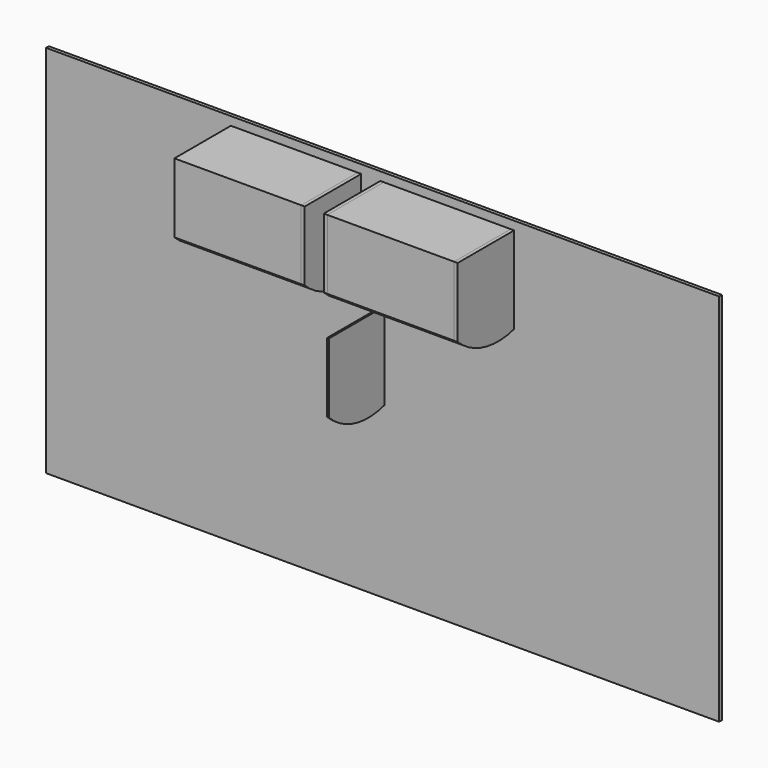
from build123d import *

# Parameters (mm, degrees)
F0_W          = 774.7
F0_H          = 431
F1_DEPTH      = 4
F3_DEPTH      = 2
F3_DEPTH_BACK = 2
F7_DEPTH      = 146
F9_DEPTH      = 2


# Not quite as in the source:
# - a pattern or mirror of a feature is missing from the dataset's text; its kind, count and spacing are read off the source's solid


with BuildPart() as f1:
    # F0 (on Front) → F1 (new body)
    with BuildSketch(Plane.XZ):
        Rectangle(F0_W, F0_H)
    extrude(amount=F1_DEPTH)

    # F8 (on Right) → F9 (join)
    with BuildSketch(Plane.YZ):
        with BuildLine():
            ThreePointArc((-83.8898100026, 0), (-46.6623748041, -21.0902592062), (-3.8898100026, -20))
            Line((-3.8898100026, -20), (-3.8898100026, 80))
            Line((-3.8898100026, 80), (-83.8898100026, 80))
            Line((-83.8898100026, 80), (-83.8898100026, 0))
        make_face()
    extrude(amount=F9_DEPTH)


with BuildPart() as f3:
    # F2 (on Right) → F3 (new body, two sides)
    with BuildSketch(Plane.YZ) as f3_sk:
        with BuildLine():
            ThreePointArc((-86.0752825102, 126.2208398572), (-48.079888449, 105.4589891292), (-4.7887346299, 106.2208398572))
            Line((-4.7887346299, 106.2208398572), (-4.7887346299, 206.2208398572))
            Line((-4.7887346299, 206.2208398572), (-86.0752825102, 206.2208398572))
            Line((-86.0752825102, 206.2208398572), (-86.0752825102, 126.2208398572))
        make_face()
    extrude(amount=F3_DEPTH)
    extrude(f3_sk.sketch, amount=-F3_DEPTH_BACK)


with BuildPart() as f3_copies_1:
    # F3_copies: instance of F3
    add(f3.part.mirror(Plane(origin=(-15, 0, 0), x_dir=(0, 0, -1), z_dir=(-1, 0, 0))))



with BuildPart() as f3_copies1_1:
    # F3_copies1: instance of F3
    add(f3.part.mirror(Plane(origin=(-13, 0, 0), x_dir=(0, 0, -1), z_dir=(-1, 0, 0))))


with BuildPart() as f3_copies2_1:
    # F3_copies2: instance of F3
    add(f3.part.mirror(Plane(origin=(-86, 0, 0), x_dir=(0, 0, -1), z_dir=(-1, 0, 0))))


with BuildPart() as f5_1:
    # F5: instance of F3
    add(f3.part.mirror(Plane.YZ.offset(75)))


with BuildPart() as f7:
    # F7 (new): a face of the model
    f7_faces = [f3.part.faces().sort_by_distance(p)[0] for p in [
        (2, -44.1296538263, 157.155690045),
    ]]
    extrude(f7_faces, amount=F7_DEPTH)


with BuildPart() as f3_copies_1_1:
    add(f3_copies_1.part)

    add(f3_copies2_1.part)  # F7_copies merges F3_copies2_1
    # F7_copies: F7 across plane
    add(f7.part.mirror(Plane(origin=(-13, 0, 0), x_dir=(0, 0, -1), z_dir=(-1, 0, 0))))


solid = Compound([f1.part, f3.part, f3_copies1_1.part, f5_1.part, f7.part, f3_copies_1_1.part])
